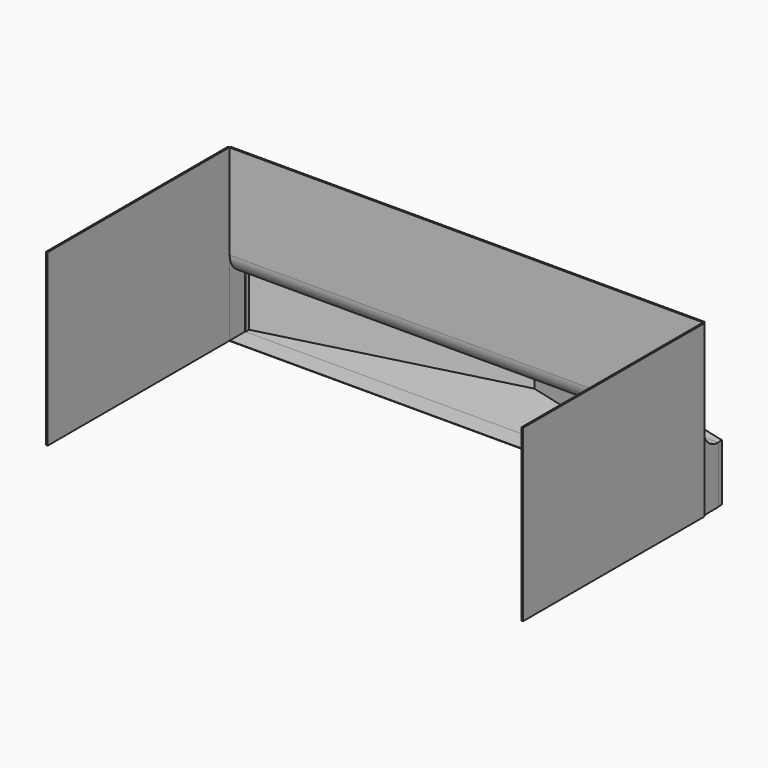
from build123d import *

# Parameters (mm, degrees)
F0_W      = 7620
F0_H      = 914.4
F1_DEPTH  = 1066.8
F3_DEPTH  = 914.401
F4_T      = -6.35
F2_R      = 457.2
F5_DEPTH  = 6.35
F7_DEPTH  = 7620
F9_DEPTH  = 6.35
F14_DEPTH = 6.35
F16_DEPTH = 25.4
F18_W     = 7632.7
F18_H     = 1524
F19_DEPTH = 25.4


# Not quite as in the source:
# - a feature of the source that left no trace in its solid (it failed there, or was rolled back) is left out
# - a pattern or mirror of a feature is missing from the dataset's text; its kind, count and spacing are read off the source's solid


with BuildPart() as f1:
    # F0 (on Front) → F1 (new body)
    with BuildSketch(Plane.XZ):
        with Locations((3810, 457.2)):
            Rectangle(F0_W, F0_H)
    extrude(amount=F1_DEPTH)

    # F2 (on face) → F3 (cut, through all)
    with BuildSketch(Plane.XY.offset(914.4)):
        Polygon((7620, 0), (3810, 0), (7620, -990.5999898911), align=None)
        Polygon((0, -990.5999898911), (3810, 0), (0, 0), align=None)
    extrude(amount=-F3_DEPTH, mode=Mode.SUBTRACT)

    # F4
    f4_openings = [f1.faces().sort_by_distance(p)[0] for p in [
        (3810, -1066.8, 457.2),
    ]]
    offset(amount=F4_T, openings=f4_openings)

    # F2 (on face) → F5 (cut, through all)
    with BuildSketch(Plane.XY.offset(914.4)):
        with Locations((3810, -533.4)):
            Circle(F2_R)
    extrude(amount=-F5_DEPTH, mode=Mode.SUBTRACT)


with BuildPart() as f7:
    # F6 (on face) → F7 (new body, through all)
    with BuildSketch(Plane.YZ.offset(7620)):
        with BuildLine():
            ThreePointArc((-1066.8, 914.4), (-1282.3261469057, 1003.6738530943), (-1371.6, 1219.2))
            Line((-1371.6, 1219.2), (-1377.95, 1219.2))
            ThreePointArc((-1377.95, 1219.2), (-1286.8162749662, 999.1837250338), (-1066.8, 908.05))
            Line((-1066.8, 908.05), (-1066.8, 914.4))
        make_face()
    extrude(amount=-F7_DEPTH)


with BuildPart() as f9:
    # F8 (on face) → F9 (new body)
    with BuildSketch(Plane.YZ.offset(7620)):
        with BuildLine():
            Line((-1371.6, 1219.2), (-1377.95, 1219.2))
            ThreePointArc((-1377.95, 1219.2), (-1286.8162749662, 999.1837250338), (-1066.8, 908.05))
            Line((-1066.8, 908.05), (-1066.8, 914.4))
            ThreePointArc((-1066.8, 914.4), (-1282.3261469057, 1003.6738530943), (-1371.6, 1219.2))
        make_face()
        with BuildLine():
            ThreePointArc((-1066.8, 908.05), (-1286.8162749662, 999.1837250338), (-1377.95, 1219.2))
            Line((-1377.95, 1219.2), (-1377.95, 0))
            Line((-1377.95, 0), (-1066.8, 0))
            Line((-1066.8, 0), (-1066.8, 908.05))
        make_face()
    extrude(amount=F9_DEPTH)


with BuildPart() as f9_copies_1:
    # F9_copies: instance of F9
    add(f9.part.mirror(Plane(origin=(3810, 0, 0), x_dir=(0, 0, -1), z_dir=(-1, 0, 0))))


with BuildPart() as f14:
    # F13 (on face) → F14 (new body)
    with BuildSketch(Plane(origin=(0, 0, 0), x_dir=(1, 0, 0), z_dir=(0, 0, -1))):
        Polygon((-6.35, 1377.95), (-6.35, 1066.8), (0, 1066.8), (7620, 1066.8), (7626.35, 1066.8), (7626.35, 1377.95), align=None)
    extrude(amount=-F14_DEPTH)


with BuildPart() as f16:
    # F15 (on face) → F16 (new body)
    with BuildSketch(Plane.YZ.offset(7626.35)):
        Polygon((-1377.95, 1219.2), (-1377.95, 2743.2), (-5035.55, 2743.2), (-5035.55, 0), (-1377.95, 0), align=None)
    extrude(amount=F16_DEPTH)


with BuildPart() as f16_copies_1:
    # F16_copies: instance of F16
    add(f16.part.mirror(Plane(origin=(3810, 0, 0), x_dir=(0, 0, -1), z_dir=(-1, 0, 0))))


with BuildPart() as f19:
    # F18 (on face) → F19 (new body)
    with BuildSketch(Plane(origin=(0, -1377.95, 0), x_dir=(-1, 0, 0), z_dir=(0, 1, 0))):
        with Locations((-3810, 1981.2)):
            Rectangle(F18_W, F18_H)
    extrude(amount=F19_DEPTH)


solid = Compound([f1.part, f7.part, f9.part, f9_copies_1.part, f14.part, f16.part, f16_copies_1.part, f19.part])
